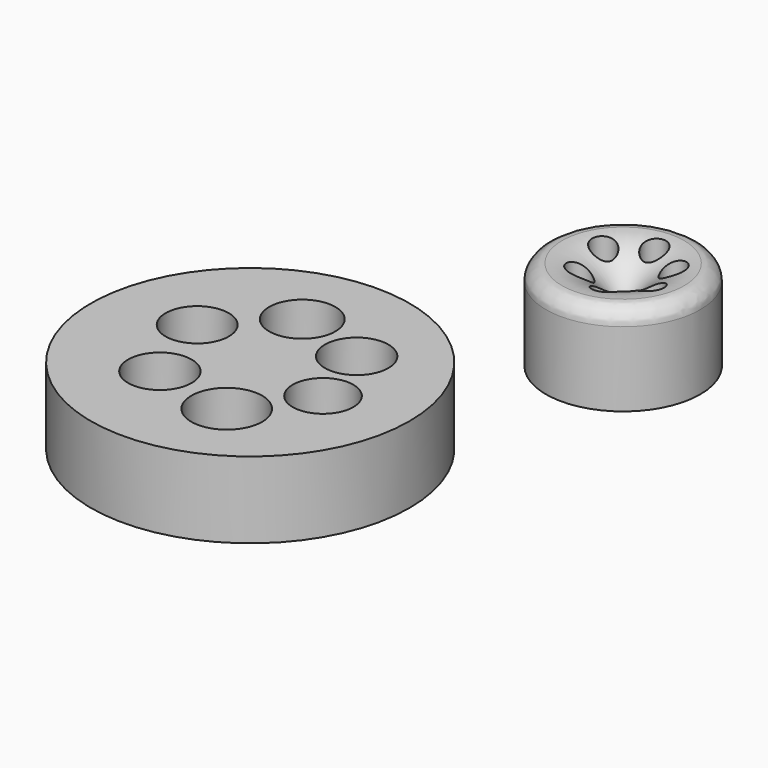
from build123d import *

# Parameters (mm, degrees)
F0_R     = 8.9744003975
F0_R_2   = 1.379335325
F0_R_3   = 0.5330047415
F1_DEPTH = 10.5156
F3_R     = 1.8396307345
F4_R     = 18.5422013788
F4_R_2   = 3.6987589535
F4_R_3   = 4.1183896775
F4_R_4   = 3.5266295723
F4_R_5   = 3.6767259014
F4_R_6   = 3.8534276879
F4_R_7   = 3.6986222034
F5_DEPTH = 8.89


# Not quite as in the source:
# - a fillet or chamfer that OpenCascade refuses, or shapes differently, is made with other operations: its cross-section is extruded or revolved along the edge and cut away or added


with BuildPart() as f1:
    # F0 (on Top) → F1 (new body)
    with BuildSketch(Plane.XY):
        with Locations((-15.7271921635, 9.9438205361)):
            Circle(F0_R)
        with Locations((-18.7826585025, 7.4001010507)):
            Circle(F0_R_2, mode=Mode.SUBTRACT)
        with Locations((-14.607205987, 5.8650835417)):
            Circle(F0_R_2, mode=Mode.SUBTRACT)
        with Locations((-11.340148747, 8.6051486433)):
            Circle(F0_R_2, mode=Mode.SUBTRACT)
        with Locations((-19.7577234358, 12.096138671)):
            Circle(F0_R_2, mode=Mode.SUBTRACT)
        with Locations((-15.8314276487, 14.6171692759)):
            Circle(F0_R_2, mode=Mode.SUBTRACT)
        with Locations((-15.7271921635, 9.9438205361)):
            Circle(F0_R_3, mode=Mode.SUBTRACT)
        with Locations((-12.0285199955, 12.6594211906)):
            Circle(F0_R_2, mode=Mode.SUBTRACT)
    extrude(amount=F1_DEPTH)

    # F2: fillet of radius 6.6839916688 on 1 edges, made by hand

    # F2_s1 → F2_t2 (revolve, cut)
    with BuildSketch(Plane.XZ.offset(-9.9438205361)):
        with BuildLine():
            ThreePointArc((-15.194187422, 3.8316083312), (-13.2364915876, 8.5579041656), (-8.5101957532, 10.5156))
            Line((-8.5101957532, 10.5156), (-15.194187422, 10.5156))
            Line((-15.194187422, 10.5156), (-15.194187422, 3.8316083312))
        make_face()
    revolve(axis=Axis((-15.7271921635, 9.9438205361, 10.5156), (0, 0, 1)), mode=Mode.SUBTRACT)

    # F3
    f3_edges = [f1.edges().sort_by_distance(p)[0] for p in [
        (-24.701593, 9.943821, 10.5156),
    ]]
    fillet(f3_edges, radius=F3_R)


with BuildPart() as f5:
    # F4 (on Top) → F5 (new body)
    with BuildSketch(Plane.XY):
        with Locations((-31.955409795, -23.9933803678)):
            Circle(F4_R)
        with Locations((-37.2521616518, -30.5015873164)):
            Circle(F4_R_2, mode=Mode.SUBTRACT)
        with Locations((-27.9033742845, -32.4668027461)):
            Circle(F4_R_3, mode=Mode.SUBTRACT)
        with Locations((-22.6526260376, -25.0338688493)):
            Circle(F4_R_4, mode=Mode.SUBTRACT)
        with Locations((-40.3158329427, -21.2480016053)):
            Circle(F4_R_5, mode=Mode.SUBTRACT)
        with Locations((-33.5527025163, -14.4228152931)):
            Circle(F4_R_6, mode=Mode.SUBTRACT)
        with Locations((-25.1316726208, -17.0435551554)):
            Circle(F4_R_7, mode=Mode.SUBTRACT)
    extrude(amount=F5_DEPTH)


solid = Compound([f1.part, f5.part])
